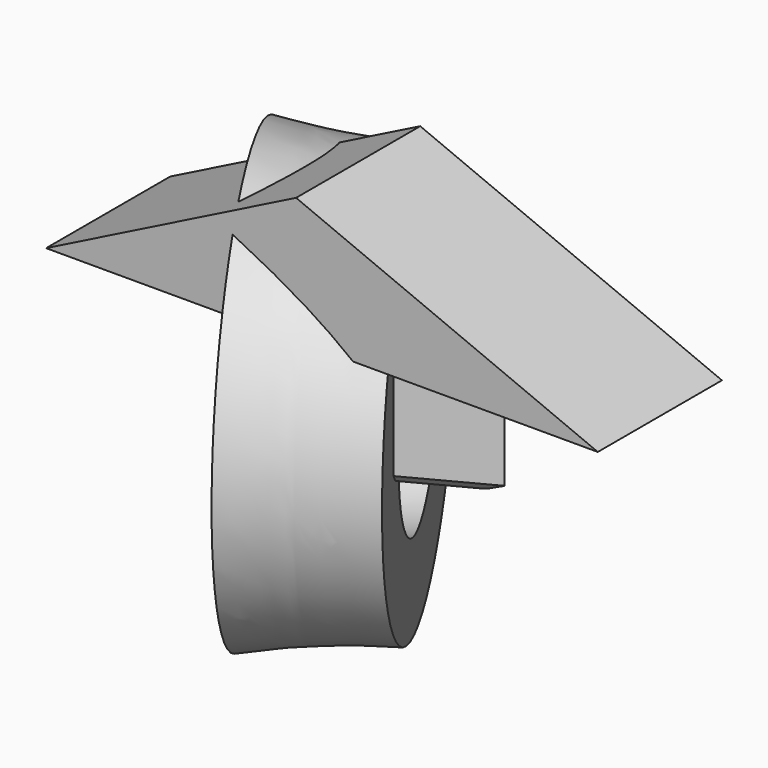
from build123d import *

# Parameters (mm, degrees)
F1_DEPTH = 73.23845
F3_DEPTH = 57.87031
F4_SIZE  = 5.08
F5_R     = 5.07999
F6_W     = 72.171472013
F6_H     = 40.1722677052


# Not quite as in the source:
# - a fillet or chamfer is up to 0.001 mm smaller than in the source, because OpenCascade refuses the exact size


with BuildPart() as f1:
    # F0 (on Front) → F1 (new body)
    with BuildSketch(Plane.XZ):
        Polygon((0, 59.2983625829), (-118.0220618844, 0), (142.4238681793, 0), align=None)
    extrude(amount=F1_DEPTH)

    # F2 (on face) → F3 (join)
    with BuildSketch(Plane(origin=(0, 0, 0), x_dir=(1, 0, 0), z_dir=(0, 0, -1))):
        Polygon((69.1764354706, 36.619225), (0, 73.23845), (0, 0), align=None)
        Polygon((0, 0), (0, 73.23845), (-63.5601058602, 36.619225), align=None)
    extrude(amount=F3_DEPTH)

    # F4
    f4_edges = [f1.edges().sort_by_distance(p)[0] for p in [
        (34.588218, -18.309613, -57.87031),
        (34.588218, -54.928838, -57.87031),
    ]]
    chamfer(f4_edges, length=F4_SIZE)

    # F5 (radius 5.08 in the source; OpenCascade refuses exactly that, so slightly less here)
    f5_edges = [f1.edges().sort_by_distance(p)[0] for p in [
        (-34.37973, -53.431071, -57.87031),
        (-34.37973, -19.807379, -57.87031),
        (26.559471, -19.807379, -57.87031),
        (26.559471, -53.431071, -57.87031),
    ]]
    fillet(f5_edges, radius=F5_R)

    # F6 (on Front) → F7 (revolve)
    with BuildSketch(Plane.XZ):
        with Locations((-36.0857360065, 20.0861338526)):
            Rectangle(F6_W, F6_H)
    revolve(axis=Axis((-31.7800580476, -18.3096154484, -52.79032), (0.8664808713, 0.4992102759, 0)))


solid = f1.part
